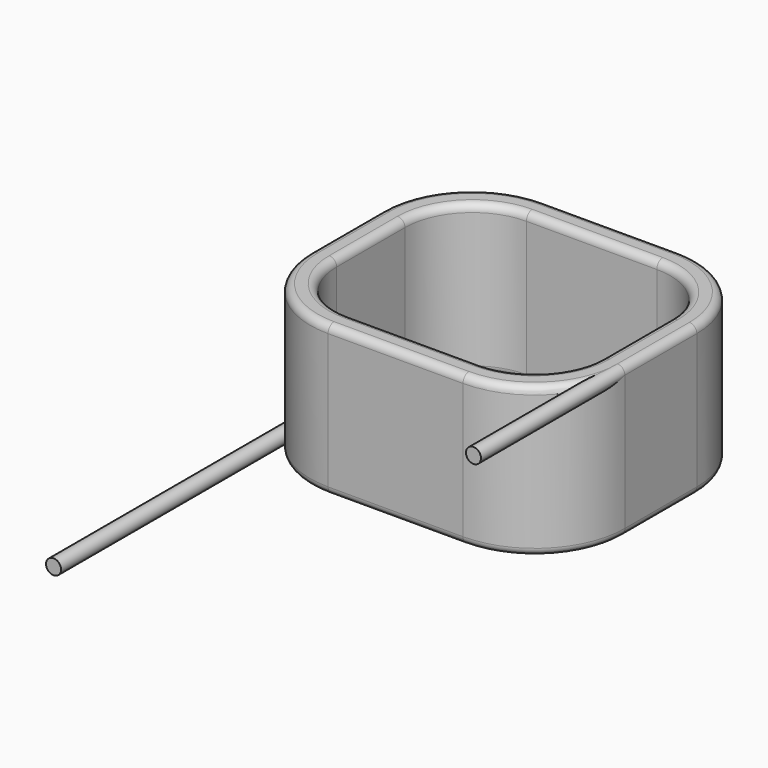
from build123d import *

# Parameters (mm, degrees)
F1_DEPTH  = 10
F3_DEPTH  = 10
F4_R      = 0.5
F5_R      = 0.1
F6_DEPTH  = 0.1
F7_R      = 0.5
F8_DEPTH  = 25
F9_R      = 0.5
F10_DEPTH = 15


# Not quite as in the source:
# - after a boolean that leaves OpenCascade's solid faulty, fix() repairs it


with BuildPart() as f1:
    # F0 (on Top) → F1 (new body)
    with BuildSketch(Plane.XY):
        with BuildLine():
            Line((-4.5, -9), (4.5, -9))
            ThreePointArc((4.5, -9), (8.7426406871, -7.2426406871), (10.5, -3))
            Line((10.5, -3), (10.5, 3))
            ThreePointArc((10.5, 3), (8.7426406871, 7.2426406871), (4.5, 9))
            Line((4.5, 9), (-4.5, 9))
            ThreePointArc((-4.5, 9), (-8.7426406871, 7.2426406871), (-10.5, 3))
            Line((-10.5, 3), (-10.5, -3))
            ThreePointArc((-10.5, -3), (-8.7426406871, -7.2426406871), (-4.5, -9))
        make_face()
    extrude(amount=F1_DEPTH)

    # F2 (on face) → F3 (cut)
    with BuildSketch(Plane.XY.offset(10)):
        with BuildLine():
            Line((-4.35, -7.35), (4.35, -7.35))
            ThreePointArc((4.35, -7.35), (7.5319805153, -6.0319805153), (8.85, -2.85))
            Line((8.85, -2.85), (8.85, 2.85))
            ThreePointArc((8.85, 2.85), (7.5319805153, 6.0319805153), (4.35, 7.35))
            Line((4.35, 7.35), (-4.35, 7.35))
            ThreePointArc((-4.35, 7.35), (-7.5319805153, 6.0319805153), (-8.85, 2.85))
            Line((-8.85, 2.85), (-8.85, -2.85))
            ThreePointArc((-8.85, -2.85), (-7.5319805153, -6.0319805153), (-4.35, -7.35))
        make_face()
    extrude(amount=-F3_DEPTH, mode=Mode.SUBTRACT)

    # F4
    f4_edges = [f1.edges().sort_by_distance(p)[0] for p in [
        (-8.742641, 7.242641, 10),
        (8.85, 0, 10),
        (-8.742641, 7.242641, 0),
        (7.531981, 6.031981, 0),
    ]]
    fillet(f4_edges, radius=F4_R)

    # F7 (on Front) → F8 (join)
    with BuildSketch(Plane.XZ):
        with Locations((-10.0158974528, 0.5172858946)):
            Circle(F7_R)
    extrude(amount=F8_DEPTH)

    # F9 (on Front) → F10 (join)
    with BuildSketch(Plane.XZ):
        with Locations((10, 9.5)):
            Circle(F9_R)
    extrude(amount=F10_DEPTH)

    add(f1.part.fix(), mode=Mode.REPLACE)


with BuildPart() as f6:
    # F5 (on Top) → F6 (new body)
    with BuildSketch(Plane.XY):
        Circle(F5_R)
    extrude(amount=F6_DEPTH)


solid = Compound([f1.part, f6.part])
